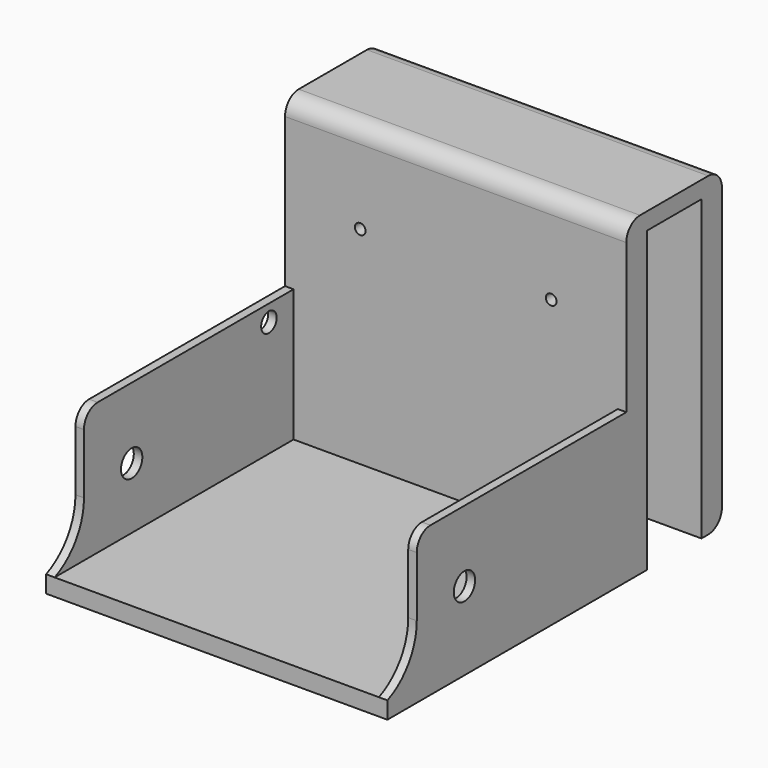
from build123d import *

# Parameters (mm, degrees)
F0_W        = 7.62
F0_H        = 88.9
F0_H_2      = 83.82
F0_W_2      = 88.9
F0_H_3      = 5.08
F1_DEPTH    = 101.6
F3_START    = 17.018
F3_DEPTH    = 78.74
F4_T1_DEPTH = 2.54
F4_T3_DEPTH = 2.54
F5_R        = 5.08
F6_R        = 5.08
F7_R        = 5.08
F8_R        = 3.9711233586
F9_DEPTH    = 154.686
F10_R       = 2.8797148657
F11_DEPTH   = 33.782
F12_R       = 1.5875
F13_DEPTH   = 85.344


# Not quite as in the source:
# - a fillet or chamfer that OpenCascade refuses, or shapes differently, is made with other operations: its cross-section is extruded or revolved along the edge and cut away or added


with BuildPart() as f1:
    # F0 (on Right) → F1 (new body)
    with BuildSketch(Plane.YZ):
        with Locations((13.97, 0)):
            Rectangle(F0_W, F0_H)
        Polygon((-10.16, 44.45), (10.16, 44.45), (17.78, 44.45), (17.78, 49.53), (-17.78, 49.53), (-17.78, 44.45), align=None)
        with Locations((-13.97, 2.54)):
            Rectangle(F0_W, F0_H_2)
        with Locations((-62.23, -41.91)):
            Rectangle(F0_W_2, F0_H_3)
        with Locations((-13.97, -41.91)):
            Rectangle(F0_W, F0_H_3)
    extrude(amount=F1_DEPTH)

    # F2 (on Front) → F3 (join)
    with BuildSketch(Plane.XZ.offset(F3_START)):
        Polygon((0, 0), (0, -39.37), (0, -44.45), (2.54, -44.45), (2.54, 0), align=None)
        Polygon((101.6, 0), (99.06, 0), (99.06, -44.45), (101.6, -44.45), (101.6, -39.37), align=None)
    extrude(amount=F3_DEPTH)

    # F4: fillet of radius 17.78 on 2 edges, made by hand

    # F4_s2 → F4_t1 (join)
    with BuildSketch(Plane.YZ.offset(99.06)):
        with BuildLine():
            ThreePointArc((-106.68, -39.37), (-98.7382763539, -32.8196066778), (-95.758, -22.9658469893))
            Line((-95.758, -22.9658469893), (-95.758, -39.37))
            Line((-95.758, -39.37), (-106.68, -39.37))
        make_face()
    extrude(amount=F4_T1_DEPTH)

    # F4_s4 → F4_t3 (join)
    with BuildSketch(Plane.YZ):
        with BuildLine():
            ThreePointArc((-106.68, -39.37), (-98.7382763539, -32.8196066778), (-95.758, -22.9658469893))
            Line((-95.758, -22.9658469893), (-95.758, -39.37))
            Line((-95.758, -39.37), (-106.68, -39.37))
        make_face()
    extrude(amount=F4_T3_DEPTH)

    # F5
    f5_edges = [f1.edges().sort_by_distance(p)[0] for p in [
        (1.27, -95.758, 0),
        (100.33, -95.758, 0),
    ]]
    fillet(f5_edges, radius=F5_R)

    # F6
    f6_edges = [f1.edges().sort_by_distance(p)[0] for p in [
        (50.8, -17.78, 49.53),
        (50.8, 17.78, 49.53),
    ]]
    fillet(f6_edges, radius=F6_R)

    # F7
    f7_edges = [f1.edges().sort_by_distance(p)[0] for p in [
        (50.8, 17.78, -44.45),
    ]]
    fillet(f7_edges, radius=F7_R)

    # F8 (on Right) → F9 (cut)
    with BuildSketch(Plane.YZ):
        with Locations((-78.0128240585, -21.108629182)):
            Circle(F8_R)
    extrude(amount=F9_DEPTH, mode=Mode.SUBTRACT)

    # F10 (on Right) → F11 (cut)
    with BuildSketch(Plane.YZ):
        with Locations((-26.9465316087, -4.8854034394)):
            Circle(F10_R)
    extrude(amount=F11_DEPTH, mode=Mode.SUBTRACT)

    # F12 (on face) → F13 (cut)
    with BuildSketch(Plane.XZ.offset(17.78)):
        with Locations((22.3786290735, 22.225)):
            Circle(F12_R)
        with Locations((79.2213709265, 22.225)):
            Circle(F12_R)
    extrude(amount=-F13_DEPTH, mode=Mode.SUBTRACT)


solid = f1.part
